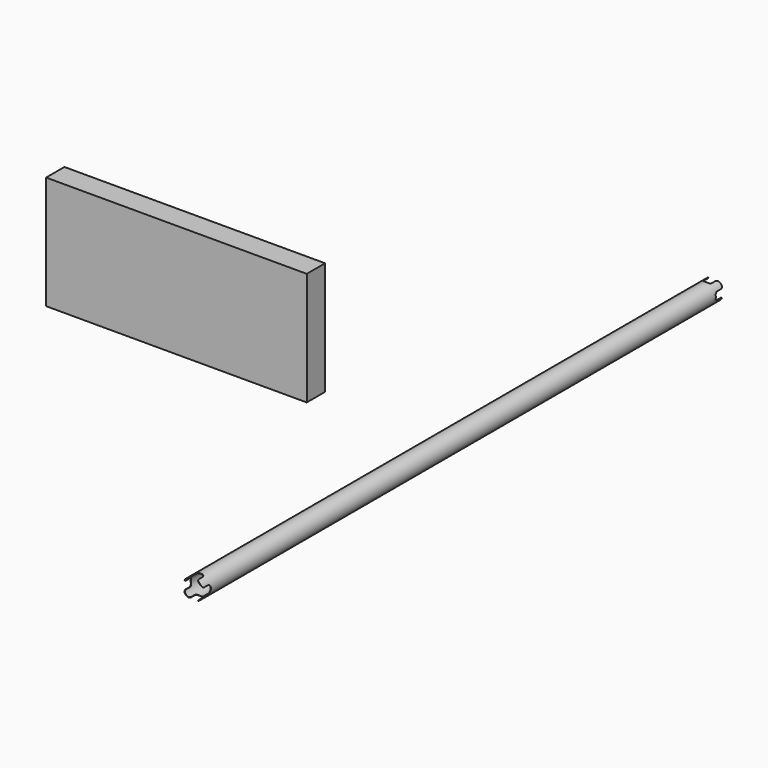
from build123d import *

# Parameters (mm, degrees)
F0_R     = 15.5
F0_R_2   = 14.95
F1_DEPTH = 1000
F3_DEPTH = 20
F5_DEPTH = 20
F6_W     = 400.5707651377
F6_H     = 35.2197885513
F7_DEPTH = 174


# Not quite as in the source:
# - a pattern or mirror of a feature is missing from the dataset's text; its kind, count and spacing are read off the source's solid


with BuildPart() as f1:
    # F0 (on Front) → F1 (new body)
    with BuildSketch(Plane.XZ):
        Circle(F0_R)
        Circle(F0_R_2, mode=Mode.SUBTRACT)
    extrude(amount=F1_DEPTH)

    # F2 (on Top) → F3 (cut, symmetric)
    with BuildSketch(Plane.XY):
        with BuildLine():
            ThreePointArc((-6, -11), (-4.8284271247, -13.8284271247), (-2, -15))
            Line((-2, -15), (2, -15))
            ThreePointArc((2, -15), (4.8284271247, -13.8284271247), (6, -11))
            Line((6, -11), (6, -4))
            ThreePointArc((6, -4), (7.1715728753, -1.1715728753), (10, 0))
            Line((10, 0), (20.7495384514, 0))
            Line((20.7495384514, 0), (6, 15))
            Line((6, 15), (-6, 15))
            Line((-6, 15), (-18.7897619456, 0))
            Line((-18.7897619456, 0), (-10, 0))
            ThreePointArc((-10, 0), (-7.1715728753, -1.1715728753), (-6, -4))
            Line((-6, -4), (-6, -11))
        make_face()
    f3 = extrude(amount=F3_DEPTH, both=True, mode=Mode.SUBTRACT)

    # F3_copies: F3 across plane
    add(f3.mirror(Plane(origin=(0, -500, 0), x_dir=(0, 0, -1), z_dir=(0, -1, 0))), mode=Mode.SUBTRACT)

    # F4 (on Right) → F5 (cut, symmetric)
    with BuildSketch(Plane.YZ):
        with BuildLine():
            ThreePointArc((-15, -2), (-13.8284271247, -4.8284271247), (-11, -6))
            Line((-11, -6), (-4, -6))
            ThreePointArc((-4, -6), (-1.1715728753, -7.1715728753), (0, -10))
            Line((0, -10), (0, -16.3496993482))
            Line((0, -16.3496993482), (30, -16.3496993482))
            Line((30, -16.3496993482), (30, 16.3496993482))
            Line((30, 16.3496993482), (0, 16.3496993482))
            Line((0, 16.3496993482), (0, 10))
            ThreePointArc((0, 10), (-1.1715728753, 7.1715728753), (-4, 6))
            Line((-4, 6), (-11, 6))
            ThreePointArc((-11, 6), (-13.8284271247, 4.8284271247), (-15, 2))
            Line((-15, 2), (-15, -2))
        make_face()
    f5 = extrude(amount=F5_DEPTH, both=True, mode=Mode.SUBTRACT)

    # F5_copies: F5 across plane
    add(f5.mirror(Plane(origin=(0, -500, 0), x_dir=(0, 0, -1), z_dir=(0, -1, 0))), mode=Mode.SUBTRACT)


with BuildPart() as f7:
    # F6 (on Top) → F7 (new body)
    with BuildSketch(Plane.XY):
        with Locations((-397.2257897258, -517.6098942757)):
            Rectangle(F6_W, F6_H)
    extrude(amount=F7_DEPTH)


solid = Compound([f1.part, f7.part])
